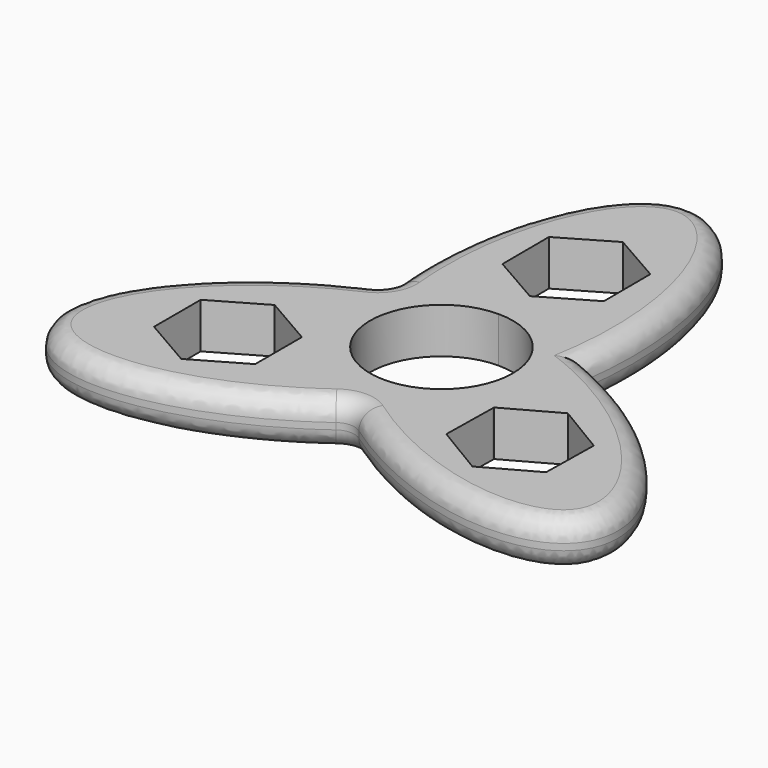
from build123d import *

# Parameters (mm, degrees)
F1_DEPTH = 7
F2_R     = 3


with BuildPart() as f1:
    # F0 (on Top) → F1 (new body)
    with BuildSketch(Plane.XY):
        with BuildLine():
            add(Edge.make_bspline(
                [(15.3449634824, 8.6599886027), (20.8857901148, 47.9699753694), (0.1382077211, 48.2294719623), (-20.6093746725, 48.4889685552), (-15.3233826686, 9.0435673342)],
                knots=[1.3004621403, 1.3004621403, 1.3004621403, 3.135231069, 3.135231069, 4.9699999977, 4.9699999977, 4.9699999977], degree=2, weights=[1, 0.6078990065, 1, 0.6078990065, 1]))
            add(Edge.make_bspline(
                [(-15.3233826686, 9.0435673342), (-52.4150402709, -5.9369646842), (-41.5139493867, -24.180924586), (-30.6128585025, -42.4248844878), (0.5209857312, -17.47341384)],
                knots=[1.3004029951, 1.3004029951, 1.3004029951, 3.1479868272, 3.1479868272, 4.9955706593, 4.9955706593, 4.9955706593], degree=2, weights=[1, 0.6027989539, 1, 0.6027989539, 1]))
            add(Edge.make_bspline(
                [(0.5209857312, -17.47341384), (31.9401455689, -41.4951398938), (41.8705229362, -23.9887355735), (51.8009003035, -6.4823312532), (15.3449634824, 8.6599886027)],
                knots=[1.3192423713, 1.3192423713, 1.3192423713, 3.1464434752, 3.1464434752, 4.9736445791, 4.9736445791, 4.9736445791], degree=2, weights=[1, 0.6108991281, 1, 0.6108991281, 1]))
        make_face()
        Polygon((-22.5166604984, -4), (-14.7224318643, -8.5), (-14.7224318643, -17.5), (-22.5166604984, -22), (-30.3108891325, -17.5), (-30.3108891325, -8.5), align=None, mode=Mode.SUBTRACT)
        with BuildLine():
            ThreePointArc((0, 11), (7.7781745931, 7.7781745931), (11, 0))
            ThreePointArc((11, 0), (-7.7781745931, -7.7781745931), (0, 11))
        make_face(mode=Mode.SUBTRACT)
        Polygon((22.6688952582, -4), (30.3870065124, -8.6318391694), (30.2347717525, -17.6318391694), (22.3644257386, -22), (14.6463144844, -17.3681608306), (14.7956045933, -8.5422462948), (14.7985492443, -8.3681608306), align=None, mode=Mode.SUBTRACT)
        Polygon((0.0371564592, 17.0000767005), (0, 17.0213249431), (-7.7755839799, 21.4678599126), (-7.8127404391, 30.4677832121), (-0.0371564592, 34.9999232995), (7.7755839799, 30.5321400874), (7.8127404391, 21.5322167879), align=None, mode=Mode.SUBTRACT)
    extrude(amount=F1_DEPTH)

    # F2
    f2_edges = [f1.edges().sort_by_distance(p)[0] for p in [
        (-41.467196, -24.258213, 7),
        (0.230732, 48.227785, 7),
        (41.906029, -23.925451, 7),
        (41.906029, -23.925451, 0),
        (-15.323383, 9.043567, 3.5),
        (0.520986, -17.473414, 3.5),
        (-41.467196, -24.258213, 0),
        (0.230732, 48.227785, 0),
    ]]
    fillet(f2_edges, radius=F2_R)


solid = f1.part
